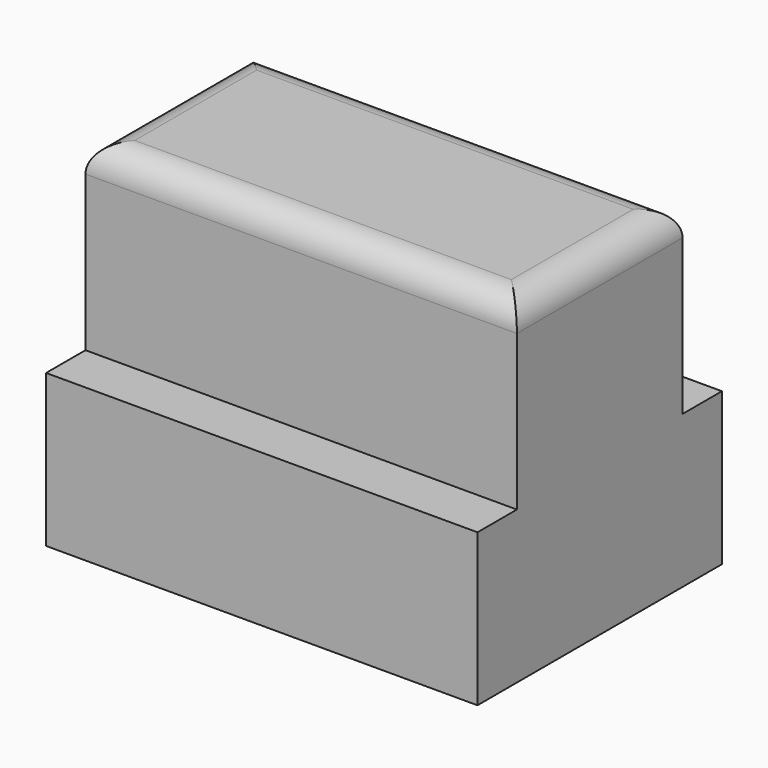
from build123d import *

# Parameters (mm, degrees)
F0_W          = 12.0142
F0_H          = 5.7658
F1_DEPTH      = 5.08
F2_W          = 12.0142
F2_H          = 8.509
F3_DEPTH      = 4.2418
F4_R          = 0.762
F6_W          = 4.1768109557
F6_H          = 2.54
F7_DEPTH      = 4.2418
F5_W          = 3.302
F5_H          = 2.54
F8_DEPTH      = 4.318
F8_DEPTH_BACK = 3.048


with BuildPart() as f1:
    # F0 (on Top) → F1 (new body)
    with BuildSketch(Plane.XY):
        Rectangle(F0_W, F0_H)
    extrude(amount=F1_DEPTH)

    # F2 (on Top) → F3 (join)
    with BuildSketch(Plane.XY):
        Rectangle(F2_W, F2_H)
    extrude(amount=-F3_DEPTH)

    # F4
    f4_edges = [f1.edges().sort_by_distance(p)[0] for p in [
        (6.0071, 0, 5.08),
        (0, 2.8829, 5.08),
        (-6.0071, 0, 5.08),
        (0, -2.8829, 5.08),
    ]]
    fillet(f4_edges, radius=F4_R)

    # F6 (on Top) → F7 (cut)
    with BuildSketch(Plane.XY):
        with Locations((-3.4931976115, 0)):
            Rectangle(F6_W, F6_H)
    extrude(amount=-F7_DEPTH, mode=Mode.SUBTRACT)

    # F5 (on Top) → F8 (cut, two sides)
    with BuildSketch(Plane.XY) as f8_sk:
        Rectangle(F5_W, F5_H)
    extrude(amount=-F8_DEPTH, mode=Mode.SUBTRACT)
    extrude(f8_sk.sketch, amount=F8_DEPTH_BACK, mode=Mode.SUBTRACT)


solid = f1.part
